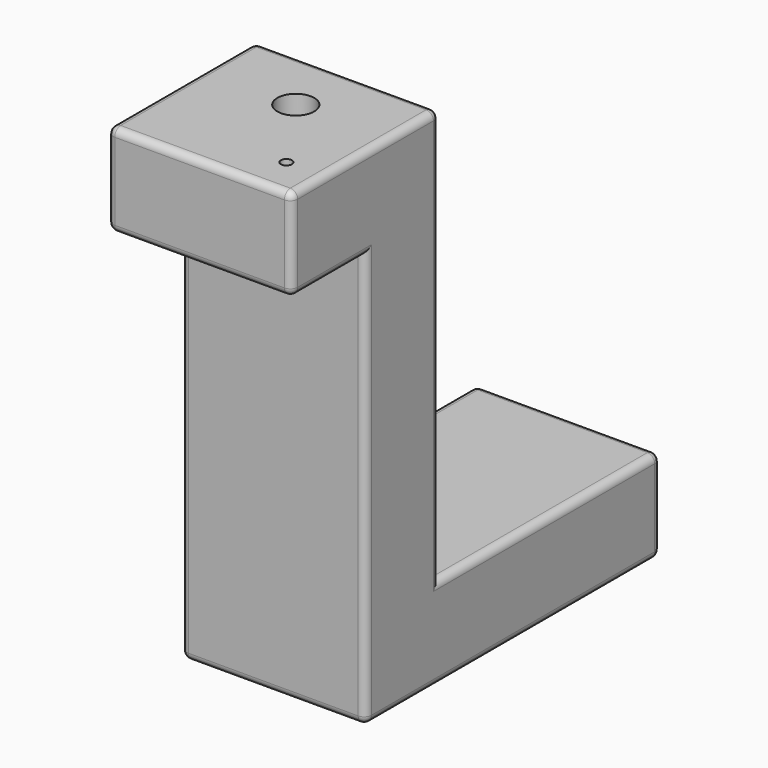
from build123d import *

# Parameters (mm, degrees)
F1_DEPTH      = 6.35
F1_DEPTH_BACK = 6.35
F2_R          = 0.508
F3_T1_DEPTH   = 7.112
F3_T3_DEPTH   = 7.62
F3_T5_DEPTH   = 28.0222646616
F3_T7_DEPTH   = 29.8002646616
F3_T9_DEPTH   = 27.94
F3_T11_DEPTH  = 20.32
F3_T13_DEPTH  = 8.89
F3_S17_W      = 0.508
F3_S17_H      = 0.508
F3_T18_DEPTH  = 0.508
F3_S23_W      = 0.508
F3_S23_H      = 0.508
F3_T24_DEPTH  = 0.508
F3_T31_DEPTH  = 8.89
F3_T35_DEPTH  = 31.0702646616
F3_T42_DEPTH  = 29.2922646616
F3_T46_DEPTH  = 21.59
F4_T1_DEPTH   = 28.0222646616
F4_T3_DEPTH   = 11.684
F4_T5_DEPTH   = 5.334
F4_T7_DEPTH   = 26.162
F4_T9_DEPTH   = 29.8002646616
F4_T11_DEPTH  = 18.542
F4_T13_DEPTH  = 7.62
F4_T15_DEPTH  = 7.112
F4_S19_W      = 0.508
F4_S19_H      = 0.508
F4_T20_DEPTH  = 0.508
F4_S25_W      = 0.508
F4_S25_H      = 0.508
F4_T26_DEPTH  = 0.508
F4_S31_W      = 0.508
F4_S31_H      = 0.508
F4_T32_DEPTH  = 0.508
F4_S37_W      = 0.508
F4_S37_H      = 0.508
F4_T38_DEPTH  = 0.508
F4_S43_W      = 0.508
F4_S43_H      = 0.508
F4_T44_DEPTH  = 0.508
F4_S49_W      = 0.508
F4_S49_H      = 0.508
F4_T50_DEPTH  = 0.508
F4_T57_DEPTH  = 19.812
F4_T61_DEPTH  = 29.2922646616
F4_T68_DEPTH  = 31.0702646616
F4_T72_DEPTH  = 8.89
F5_T1_DEPTH   = 11.684
F5_S5_W       = 0.508
F5_S5_H       = 0.508
F5_T6_DEPTH   = 0.508
F5_S11_W      = 0.508
F5_S11_H      = 0.508
F5_T12_DEPTH  = 0.508
F6_T1_DEPTH   = 11.684
F6_S5_W       = 0.508
F6_S5_H       = 0.508
F6_T6_DEPTH   = 0.508
F6_S11_W      = 0.508
F6_S11_H      = 0.508
F6_T12_DEPTH  = 0.508
F8_D          = 2.54
F8_DEPTH      = 3.175
F8_TIP        = 0.7630929862
F10_D         = 0.762


# Not quite as in the source:
# - a fillet or chamfer that OpenCascade refuses, or shapes differently, is made with other operations: its cross-section is extruded or revolved along the edge and cut away or added


with BuildPart() as f1:
    # F0 (on Right) → F1 (new body, two sides)
    with BuildSketch(Plane.YZ) as f1_sk:
        Polygon((-10.7051408962, 24.1749497761), (-23.4051408962, 24.1749497761), (-23.4051408962, 17.8249497761), (-17.0551408962, 17.8249497761), (-17.0551408962, -10.7053148855), (8.3448591038, -10.7053148855), (8.3448591038, -4.3553148855), (-10.7051408962, -4.3553148855), align=None)
    extrude(amount=F1_DEPTH)
    extrude(f1_sk.sketch, amount=-F1_DEPTH_BACK)

    # F2
    f2_edges = [f1.edges().sort_by_distance(p)[0] for p in [
        (0, -23.405141, 24.17495),
        (6.35, -17.055141, 24.17495),
        (0, -10.705141, 24.17495),
        (-6.35, -17.055141, 24.17495),
    ]]
    fillet(f2_edges, radius=F2_R)

    # F3: fillet of radius 0.508 on 7 edges, made by hand

    # F3_s2 → F3_t1 (cut)
    with BuildSketch(Plane.XY.offset(16.5549497761)):
        with BuildLine():
            ThreePointArc((6.35, -22.8971408962), (6.2012102448, -23.256351141), (5.842, -23.4051408962))
            Line((5.842, -23.4051408962), (6.35, -23.4051408962))
            Line((6.35, -23.4051408962), (6.35, -22.8971408962))
        make_face()
    extrude(amount=F3_T1_DEPTH, mode=Mode.SUBTRACT)

    # F3_s4 → F3_t3 (cut)
    with BuildSketch(Plane.XZ.offset(17.0551408962)):
        with BuildLine():
            ThreePointArc((6.35, 18.3329497761), (6.2012102448, 17.9737395313), (5.842, 17.8249497761))
            Line((5.842, 17.8249497761), (6.35, 17.8249497761))
            Line((6.35, 17.8249497761), (6.35, 18.3329497761))
        make_face()
    extrude(amount=F3_T3_DEPTH, mode=Mode.SUBTRACT)

    # F3_s6 → F3_t5 (cut)
    with BuildSketch(Plane.XY.offset(-4.3553148855)):
        with BuildLine():
            ThreePointArc((5.842, -10.7051408962), (6.2012102448, -10.8539306514), (6.35, -11.2131408962))
            Line((6.35, -11.2131408962), (6.35, -10.7051408962))
            Line((6.35, -10.7051408962), (5.842, -10.7051408962))
        make_face()
    extrude(amount=F3_T5_DEPTH, mode=Mode.SUBTRACT)

    # F3_s8 → F3_t7 (cut)
    with BuildSketch(Plane.XY.offset(-11.9753148855)):
        with BuildLine():
            ThreePointArc((6.35, -16.5471408962), (6.2012102448, -16.906351141), (5.842, -17.0551408962))
            Line((5.842, -17.0551408962), (6.35, -17.0551408962))
            Line((6.35, -17.0551408962), (6.35, -16.5471408962))
        make_face()
    extrude(amount=F3_T7_DEPTH, mode=Mode.SUBTRACT)

    # F3_s10 → F3_t9 (cut)
    with BuildSketch(Plane.XZ.offset(-9.6148591038)):
        with BuildLine():
            ThreePointArc((6.35, -10.1973148855), (6.2012102448, -10.5565251304), (5.842, -10.7053148855))
            Line((5.842, -10.7053148855), (6.35, -10.7053148855))
            Line((6.35, -10.7053148855), (6.35, -10.1973148855))
        make_face()
    extrude(amount=F3_T9_DEPTH, mode=Mode.SUBTRACT)

    # F3_s12 → F3_t11 (cut)
    with BuildSketch(Plane.XZ.offset(-9.6148591038)):
        with BuildLine():
            ThreePointArc((6.35, -4.8633148855), (6.2012102448, -4.5041046407), (5.842, -4.3553148855))
            Line((5.842, -4.3553148855), (6.35, -4.3553148855))
            Line((6.35, -4.3553148855), (6.35, -4.8633148855))
        make_face()
    extrude(amount=F3_T11_DEPTH, mode=Mode.SUBTRACT)

    # F3_s14 → F3_t13 (cut)
    with BuildSketch(Plane.XY.offset(-11.9753148855)):
        with BuildLine():
            ThreePointArc((6.35, 7.8368591038), (6.2012102448, 8.1960693486), (5.842, 8.3448591038))
            Line((5.842, 8.3448591038), (6.35, 8.3448591038))
            Line((6.35, 8.3448591038), (6.35, 7.8368591038))
        make_face()
    extrude(amount=F3_T13_DEPTH, mode=Mode.SUBTRACT)


with BuildPart() as f3_tool16:
    # F3_s17 → F3_t18 (new body)
    with BuildSketch(Plane.XZ.offset(11.2131408962)):
        with Locations((6.096, 23.9209497761)):
            Rectangle(F3_S17_W, F3_S17_H)
    extrude(amount=-F3_T18_DEPTH)

    # F3_s19 → F3_t20 (revolve, cut)
    with BuildSketch(Plane(origin=(5.842, -11.2131408962, 23.6669497761), x_dir=(-0.7071067812, 0, -0.7071067812), z_dir=(0.7071067812, 0, -0.7071067812))):
        with BuildLine():
            ThreePointArc((0, -0.508), (0.508, 0), (0, 0.508))
            Line((0, 0.508), (0, -0.508))
        make_face()
    revolve(axis=Axis((5.842, -11.2131408962, 23.6669497761), (0, 1, 0)), mode=Mode.SUBTRACT)


with BuildPart() as f1_1:
    add(f1.part)

    # F3_t15: cut F3_tool16
    add(f3_tool16.part, mode=Mode.SUBTRACT)


with BuildPart() as f3_tool22:
    # F3_s23 → F3_t24 (new body)
    with BuildSketch(Plane.YZ.offset(5.842)):
        with Locations((-23.1511408962, 23.9209497761)):
            Rectangle(F3_S23_W, F3_S23_H)
    extrude(amount=F3_T24_DEPTH)

    # F3_s25 → F3_t26 (revolve, cut)
    with BuildSketch(Plane(origin=(5.842, -22.8971408962, 23.6669497761), x_dir=(0, 0.7071067812, -0.7071067812), z_dir=(0, -0.7071067812, -0.7071067812))):
        with BuildLine():
            ThreePointArc((0, -0.508), (0.508, 0), (0, 0.508))
            Line((0, 0.508), (0, -0.508))
        make_face()
    revolve(axis=Axis((5.842, -22.8971408962, 23.6669497761), (1, 0, 0)), mode=Mode.SUBTRACT)


with BuildPart() as f1_2:
    add(f1_1.part)

    # F3_t21: cut F3_tool22
    add(f3_tool22.part, mode=Mode.SUBTRACT)


with BuildPart() as f3_tool29:
    # F3_s30 → F3_t31 (new body)
    with BuildSketch(Plane.XZ.offset(24.6751408962)):
        with BuildLine():
            ThreePointArc((6.35, 18.3329497761), (6.2012102448, 17.9737395313), (5.842, 17.8249497761))
            Line((5.842, 17.8249497761), (6.35, 17.8249497761))
            Line((6.35, 17.8249497761), (6.35, 18.3329497761))
        make_face()
    extrude(amount=-F3_T31_DEPTH)

    split(bisect_by=Plane.XZ.offset(17.0551408962), keep=Keep.BOTTOM)


with BuildPart() as f3_tool33:
    # F3_s34 → F3_t35 (new body)
    with BuildSketch(Plane.XY.offset(19.0949497761)):
        with BuildLine():
            ThreePointArc((6.35, -16.5471408962), (6.2012102448, -16.906351141), (5.842, -17.0551408962))
            Line((5.842, -17.0551408962), (6.35, -17.0551408962))
            Line((6.35, -17.0551408962), (6.35, -16.5471408962))
        make_face()
    extrude(amount=-F3_T35_DEPTH)

    split(bisect_by=Plane.XY.offset(17.8249497761), keep=Keep.TOP)


with BuildPart() as f3_tool29_1:
    add(f3_tool29.part)

    # F3_t37: intersect F3_tool33
    add(f3_tool33.part, mode=Mode.INTERSECT)


with BuildPart() as f1_3:
    add(f1_2.part)

    # F3_t27: cut F3_tool29
    add(f3_tool29_1.part, mode=Mode.SUBTRACT)


with BuildPart() as f3_tool40:
    # F3_s41 → F3_t42 (new body)
    with BuildSketch(Plane.XY.offset(-5.6253148855)):
        with BuildLine():
            ThreePointArc((5.842, -10.7051408962), (6.2012102448, -10.8539306514), (6.35, -11.2131408962))
            Line((6.35, -11.2131408962), (6.35, -10.7051408962))
            Line((6.35, -10.7051408962), (5.842, -10.7051408962))
        make_face()
    extrude(amount=F3_T42_DEPTH)

    split(bisect_by=Plane.XY.offset(-4.3553148855), keep=Keep.BOTTOM)


with BuildPart() as f3_tool44:
    # F3_s45 → F3_t46 (new body)
    with BuildSketch(Plane.XZ.offset(-9.6148591038)):
        with BuildLine():
            ThreePointArc((6.35, -4.8633148855), (6.2012102448, -4.5041046407), (5.842, -4.3553148855))
            Line((5.842, -4.3553148855), (6.35, -4.3553148855))
            Line((6.35, -4.3553148855), (6.35, -4.8633148855))
        make_face()
    extrude(amount=F3_T46_DEPTH)

    split(bisect_by=Plane.XZ.offset(10.7051408962), keep=Keep.TOP)


with BuildPart() as f3_tool40_1:
    add(f3_tool40.part)

    # F3_t48: intersect F3_tool44
    add(f3_tool44.part, mode=Mode.INTERSECT)


with BuildPart() as f1_4:
    add(f1_3.part)

    # F3_t38: cut F3_tool40
    add(f3_tool40_1.part, mode=Mode.SUBTRACT)

    # F4: fillet of radius 0.508 on 9 edges, made by hand

    # F4_s2 → F4_t1 (cut)
    with BuildSketch(Plane.XY.offset(-4.3553148855)):
        with BuildLine():
            ThreePointArc((-5.842, -10.7051408962), (-6.2012102448, -10.8539306514), (-6.35, -11.2131408962))
            Line((-6.35, -11.2131408962), (-6.35, -10.7051408962))
            Line((-6.35, -10.7051408962), (-5.842, -10.7051408962))
        make_face()
    extrude(amount=F4_T1_DEPTH, mode=Mode.SUBTRACT)

    # F4_s4 → F4_t3 (cut)
    with BuildSketch(Plane.YZ.offset(-5.842)):
        with BuildLine():
            ThreePointArc((7.8368591038, -4.3553148855), (8.1960693486, -4.5041046407), (8.3448591038, -4.8633148855))
            Line((8.3448591038, -4.8633148855), (8.3448591038, -4.3553148855))
            Line((8.3448591038, -4.3553148855), (7.8368591038, -4.3553148855))
        make_face()
        with BuildLine():
            ThreePointArc((7.8368591038, -10.7053148855), (8.1960693486, -10.5565251304), (8.3448591038, -10.1973148855))
            Line((8.3448591038, -10.1973148855), (8.3448591038, -10.7053148855))
            Line((8.3448591038, -10.7053148855), (7.8368591038, -10.7053148855))
        make_face()
    extrude(amount=F4_T3_DEPTH, mode=Mode.SUBTRACT)

    # F4_s6 → F4_t5 (cut)
    with BuildSketch(Plane.XY.offset(-10.1973148855)):
        with BuildLine():
            ThreePointArc((-6.35, 7.8368591038), (-6.2012102448, 8.1960693486), (-5.842, 8.3448591038))
            Line((-5.842, 8.3448591038), (-6.35, 8.3448591038))
            Line((-6.35, 8.3448591038), (-6.35, 7.8368591038))
        make_face()
    extrude(amount=F4_T5_DEPTH, mode=Mode.SUBTRACT)

    # F4_s8 → F4_t7 (cut)
    with BuildSketch(Plane.XZ.offset(-7.8368591038)):
        with BuildLine():
            ThreePointArc((-5.842, -10.7053148855), (-6.2012102448, -10.5565251304), (-6.35, -10.1973148855))
            Line((-6.35, -10.1973148855), (-6.35, -10.7053148855))
            Line((-6.35, -10.7053148855), (-5.842, -10.7053148855))
        make_face()
    extrude(amount=F4_T7_DEPTH, mode=Mode.SUBTRACT)

    # F4_s10 → F4_t9 (cut)
    with BuildSketch(Plane.XY.offset(-11.9753148855)):
        with BuildLine():
            ThreePointArc((-5.842, -17.0551408962), (-6.2012102448, -16.906351141), (-6.35, -16.5471408962))
            Line((-6.35, -16.5471408962), (-6.35, -17.0551408962))
            Line((-6.35, -17.0551408962), (-5.842, -17.0551408962))
        make_face()
    extrude(amount=F4_T9_DEPTH, mode=Mode.SUBTRACT)

    # F4_s12 → F4_t11 (cut)
    with BuildSketch(Plane.XZ.offset(-7.8368591038)):
        with BuildLine():
            ThreePointArc((-5.842, -4.3553148855), (-6.2012102448, -4.5041046407), (-6.35, -4.8633148855))
            Line((-6.35, -4.8633148855), (-6.35, -4.3553148855))
            Line((-6.35, -4.3553148855), (-5.842, -4.3553148855))
        make_face()
    extrude(amount=F4_T11_DEPTH, mode=Mode.SUBTRACT)

    # F4_s14 → F4_t13 (cut)
    with BuildSketch(Plane.XZ.offset(17.0551408962)):
        with BuildLine():
            ThreePointArc((-5.842, 17.8249497761), (-6.2012102448, 17.9737395313), (-6.35, 18.3329497761))
            Line((-6.35, 18.3329497761), (-6.35, 17.8249497761))
            Line((-6.35, 17.8249497761), (-5.842, 17.8249497761))
        make_face()
    extrude(amount=F4_T13_DEPTH, mode=Mode.SUBTRACT)

    # F4_s16 → F4_t15 (cut)
    with BuildSketch(Plane.XY.offset(16.5549497761)):
        with BuildLine():
            ThreePointArc((-5.842, -23.4051408962), (-6.2012102448, -23.256351141), (-6.35, -22.8971408962))
            Line((-6.35, -22.8971408962), (-6.35, -23.4051408962))
            Line((-6.35, -23.4051408962), (-5.842, -23.4051408962))
        make_face()
    extrude(amount=F4_T15_DEPTH, mode=Mode.SUBTRACT)


with BuildPart() as f4_tool18:
    # F4_s19 → F4_t20 (new body)
    with BuildSketch(Plane.XZ.offset(22.8971408962)):
        with Locations((-6.096, 23.9209497761)):
            Rectangle(F4_S19_W, F4_S19_H)
    extrude(amount=F4_T20_DEPTH)

    # F4_s21 → F4_t22 (revolve, cut)
    with BuildSketch(Plane(origin=(-5.842, -22.8971408962, 23.6669497761), x_dir=(0.7071067812, 0, -0.7071067812), z_dir=(-0.7071067812, 0, -0.7071067812))):
        with BuildLine():
            ThreePointArc((0, -0.508), (0.508, 0), (0, 0.508))
            Line((0, 0.508), (0, -0.508))
        make_face()
    revolve(axis=Axis((-5.842, -22.8971408962, 23.6669497761), (0, -1, 0)), mode=Mode.SUBTRACT)


with BuildPart() as f1_5:
    add(f1_4.part)

    # F4_t17: cut F4_tool18
    add(f4_tool18.part, mode=Mode.SUBTRACT)


with BuildPart() as f4_tool24:
    # F4_s25 → F4_t26 (new body)
    with BuildSketch(Plane.XY.offset(-10.1973148855)):
        with Locations((6.096, 8.0908591038)):
            Rectangle(F4_S25_W, F4_S25_H)
    extrude(amount=-F4_T26_DEPTH)

    # F4_s27 → F4_t28 (revolve, cut)
    with BuildSketch(Plane(origin=(5.842, 7.8368591038, -10.1973148855), x_dir=(-0.7071067812, -0.7071067812, 0), z_dir=(0.7071067812, -0.7071067812, 0))):
        with BuildLine():
            ThreePointArc((0, -0.508), (0.508, 0), (0, 0.508))
            Line((0, 0.508), (0, -0.508))
        make_face()
    revolve(axis=Axis((5.842, 7.8368591038, -10.1973148855), (0, 0, -1)), mode=Mode.SUBTRACT)


with BuildPart() as f1_6:
    add(f1_5.part)

    # F4_t23: cut F4_tool24
    add(f4_tool24.part, mode=Mode.SUBTRACT)


with BuildPart() as f4_tool30:
    # F4_s31 → F4_t32 (new body)
    with BuildSketch(Plane.XY.offset(-4.8633148855)):
        with Locations((6.096, 8.0908591038)):
            Rectangle(F4_S31_W, F4_S31_H)
    extrude(amount=F4_T32_DEPTH)

    # F4_s33 → F4_t34 (revolve, cut)
    with BuildSketch(Plane(origin=(5.842, 7.8368591038, -4.8633148855), x_dir=(-0.7071067812, -0.7071067812, 0), z_dir=(-0.7071067812, 0.7071067812, 0))):
        with BuildLine():
            ThreePointArc((0, -0.508), (0.508, 0), (0, 0.508))
            Line((0, 0.508), (0, -0.508))
        make_face()
    revolve(axis=Axis((5.842, 7.8368591038, -4.8633148855), (0, 0, 1)), mode=Mode.SUBTRACT)


with BuildPart() as f1_7:
    add(f1_6.part)

    # F4_t29: cut F4_tool30
    add(f4_tool30.part, mode=Mode.SUBTRACT)


with BuildPart() as f4_tool36:
    # F4_s37 → F4_t38 (new body)
    with BuildSketch(Plane.XZ.offset(11.2131408962)):
        with Locations((-6.096, 23.9209497761)):
            Rectangle(F4_S37_W, F4_S37_H)
    extrude(amount=-F4_T38_DEPTH)

    # F4_s39 → F4_t40 (revolve, cut)
    with BuildSketch(Plane(origin=(-5.842, -11.2131408962, 23.6669497761), x_dir=(0.7071067812, 0, -0.7071067812), z_dir=(0.7071067812, 0, 0.7071067812))):
        with BuildLine():
            ThreePointArc((0, -0.508), (0.508, 0), (0, 0.508))
            Line((0, 0.508), (0, -0.508))
        make_face()
    revolve(axis=Axis((-5.842, -11.2131408962, 23.6669497761), (0, 1, 0)), mode=Mode.SUBTRACT)


with BuildPart() as f1_8:
    add(f1_7.part)

    # F4_t35: cut F4_tool36
    add(f4_tool36.part, mode=Mode.SUBTRACT)


with BuildPart() as f4_tool42:
    # F4_s43 → F4_t44 (new body)
    with BuildSketch(Plane.XY.offset(-4.8633148855)):
        with Locations((-6.096, 8.0908591038)):
            Rectangle(F4_S43_W, F4_S43_H)
    extrude(amount=F4_T44_DEPTH)

    # F4_s45 → F4_t46 (revolve, cut)
    with BuildSketch(Plane(origin=(-5.842, 7.8368591038, -4.8633148855), x_dir=(0.7071067812, -0.7071067812, 0), z_dir=(-0.7071067812, -0.7071067812, 0))):
        with BuildLine():
            ThreePointArc((0, -0.508), (0.508, 0), (0, 0.508))
            Line((0, 0.508), (0, -0.508))
        make_face()
    revolve(axis=Axis((-5.842, 7.8368591038, -4.8633148855), (0, 0, 1)), mode=Mode.SUBTRACT)


with BuildPart() as f1_9:
    add(f1_8.part)

    # F4_t41: cut F4_tool42
    add(f4_tool42.part, mode=Mode.SUBTRACT)


with BuildPart() as f4_tool48:
    # F4_s49 → F4_t50 (new body)
    with BuildSketch(Plane.XY.offset(-10.1973148855)):
        with Locations((-6.096, 8.0908591038)):
            Rectangle(F4_S49_W, F4_S49_H)
    extrude(amount=-F4_T50_DEPTH)

    # F4_s51 → F4_t52 (revolve, cut)
    with BuildSketch(Plane(origin=(-5.842, 7.8368591038, -10.1973148855), x_dir=(0.7071067812, -0.7071067812, 0), z_dir=(0.7071067812, 0.7071067812, 0))):
        with BuildLine():
            ThreePointArc((0, -0.508), (0.508, 0), (0, 0.508))
            Line((0, 0.508), (0, -0.508))
        make_face()
    revolve(axis=Axis((-5.842, 7.8368591038, -10.1973148855), (0, 0, -1)), mode=Mode.SUBTRACT)


with BuildPart() as f1_10:
    add(f1_9.part)

    # F4_t47: cut F4_tool48
    add(f4_tool48.part, mode=Mode.SUBTRACT)


with BuildPart() as f4_tool55:
    # F4_s56 → F4_t57 (new body)
    with BuildSketch(Plane.XZ.offset(-7.8368591038)):
        with BuildLine():
            ThreePointArc((-5.842, -4.3553148855), (-6.2012102448, -4.5041046407), (-6.35, -4.8633148855))
            Line((-6.35, -4.8633148855), (-6.35, -4.3553148855))
            Line((-6.35, -4.3553148855), (-5.842, -4.3553148855))
        make_face()
    extrude(amount=F4_T57_DEPTH)

    split(bisect_by=Plane.XZ.offset(10.7051408962), keep=Keep.TOP)


with BuildPart() as f4_tool59:
    # F4_s60 → F4_t61 (new body)
    with BuildSketch(Plane.XY.offset(-5.6253148855)):
        with BuildLine():
            ThreePointArc((-5.842, -10.7051408962), (-6.2012102448, -10.8539306514), (-6.35, -11.2131408962))
            Line((-6.35, -11.2131408962), (-6.35, -10.7051408962))
            Line((-6.35, -10.7051408962), (-5.842, -10.7051408962))
        make_face()
    extrude(amount=F4_T61_DEPTH)

    split(bisect_by=Plane.XY.offset(-4.3553148855), keep=Keep.BOTTOM)


with BuildPart() as f4_tool55_1:
    add(f4_tool55.part)

    # F4_t63: intersect F4_tool59
    add(f4_tool59.part, mode=Mode.INTERSECT)


with BuildPart() as f1_11:
    add(f1_10.part)

    # F4_t53: cut F4_tool55
    add(f4_tool55_1.part, mode=Mode.SUBTRACT)


with BuildPart() as f4_tool66:
    # F4_s67 → F4_t68 (new body)
    with BuildSketch(Plane.XY.offset(19.0949497761)):
        with BuildLine():
            ThreePointArc((-5.842, -17.0551408962), (-6.2012102448, -16.906351141), (-6.35, -16.5471408962))
            Line((-6.35, -16.5471408962), (-6.35, -17.0551408962))
            Line((-6.35, -17.0551408962), (-5.842, -17.0551408962))
        make_face()
    extrude(amount=-F4_T68_DEPTH)

    split(bisect_by=Plane.XY.offset(17.8249497761), keep=Keep.TOP)


with BuildPart() as f4_tool70:
    # F4_s71 → F4_t72 (new body)
    with BuildSketch(Plane.XZ.offset(24.6751408962)):
        with BuildLine():
            ThreePointArc((-5.842, 17.8249497761), (-6.2012102448, 17.9737395313), (-6.35, 18.3329497761))
            Line((-6.35, 18.3329497761), (-6.35, 17.8249497761))
            Line((-6.35, 17.8249497761), (-5.842, 17.8249497761))
        make_face()
    extrude(amount=-F4_T72_DEPTH)

    split(bisect_by=Plane.XZ.offset(17.0551408962), keep=Keep.BOTTOM)


with BuildPart() as f4_tool66_1:
    add(f4_tool66.part)

    # F4_t74: intersect F4_tool70
    add(f4_tool70.part, mode=Mode.INTERSECT)


with BuildPart() as f1_12:
    add(f1_11.part)

    # F4_t64: cut F4_tool66
    add(f4_tool66_1.part, mode=Mode.SUBTRACT)

    # F5: fillet of radius 0.508 on 1 edges, made by hand

    # F5_s2 → F5_t1 (cut)
    with BuildSketch(Plane.YZ.offset(-5.842)):
        with BuildLine():
            ThreePointArc((-17.0551408962, -10.1973148855), (-16.906351141, -10.5565251304), (-16.5471408962, -10.7053148855))
            Line((-16.5471408962, -10.7053148855), (-17.0551408962, -10.7053148855))
            Line((-17.0551408962, -10.7053148855), (-17.0551408962, -10.1973148855))
        make_face()
    extrude(amount=F5_T1_DEPTH, mode=Mode.SUBTRACT)


with BuildPart() as f5_tool4:
    # F5_s5 → F5_t6 (new body)
    with BuildSketch(Plane.XZ.offset(16.5471408962)):
        with Locations((-6.096, -10.4513148855)):
            Rectangle(F5_S5_W, F5_S5_H)
    extrude(amount=F5_T6_DEPTH)

    # F5_s7 → F5_t8 (revolve, cut)
    with BuildSketch(Plane(origin=(-5.842, -16.5471408962, -10.1973148855), x_dir=(0.7071067812, 0, 0.7071067812), z_dir=(0.7071067812, 0, -0.7071067812))):
        with BuildLine():
            ThreePointArc((0, -0.508), (0.508, 0), (0, 0.508))
            Line((0, 0.508), (0, -0.508))
        make_face()
    revolve(axis=Axis((-5.842, -16.5471408962, -10.1973148855), (0, -1, 0)), mode=Mode.SUBTRACT)


with BuildPart() as f1_13:
    add(f1_12.part)

    # F5_t3: cut F5_tool4
    add(f5_tool4.part, mode=Mode.SUBTRACT)


with BuildPart() as f5_tool10:
    # F5_s11 → F5_t12 (new body)
    with BuildSketch(Plane.XZ.offset(16.5471408962)):
        with Locations((6.096, -10.4513148855)):
            Rectangle(F5_S11_W, F5_S11_H)
    extrude(amount=F5_T12_DEPTH)

    # F5_s13 → F5_t14 (revolve, cut)
    with BuildSketch(Plane(origin=(5.842, -16.5471408962, -10.1973148855), x_dir=(-0.7071067812, 0, 0.7071067812), z_dir=(0.7071067812, 0, 0.7071067812))):
        with BuildLine():
            ThreePointArc((0, -0.508), (0.508, 0), (0, 0.508))
            Line((0, 0.508), (0, -0.508))
        make_face()
    revolve(axis=Axis((5.842, -16.5471408962, -10.1973148855), (0, -1, 0)), mode=Mode.SUBTRACT)


with BuildPart() as f1_14:
    add(f1_13.part)

    # F5_t9: cut F5_tool10
    add(f5_tool10.part, mode=Mode.SUBTRACT)

    # F6: fillet of radius 0.508 on 1 edges, made by hand

    # F6_s2 → F6_t1 (cut)
    with BuildSketch(Plane.YZ.offset(-5.842)):
        with BuildLine():
            ThreePointArc((-23.4051408962, 18.3329497761), (-23.256351141, 17.9737395313), (-22.8971408962, 17.8249497761))
            Line((-22.8971408962, 17.8249497761), (-23.4051408962, 17.8249497761))
            Line((-23.4051408962, 17.8249497761), (-23.4051408962, 18.3329497761))
        make_face()
    extrude(amount=F6_T1_DEPTH, mode=Mode.SUBTRACT)


with BuildPart() as f6_tool4:
    # F6_s5 → F6_t6 (new body)
    with BuildSketch(Plane.XZ.offset(22.8971408962)):
        with Locations((-6.096, 18.0789497761)):
            Rectangle(F6_S5_W, F6_S5_H)
    extrude(amount=F6_T6_DEPTH)

    # F6_s7 → F6_t8 (revolve, cut)
    with BuildSketch(Plane(origin=(-5.842, -22.8971408962, 18.3329497761), x_dir=(0.7071067812, 0, 0.7071067812), z_dir=(0.7071067812, 0, -0.7071067812))):
        with BuildLine():
            ThreePointArc((0, -0.508), (0.508, 0), (0, 0.508))
            Line((0, 0.508), (0, -0.508))
        make_face()
    revolve(axis=Axis((-5.842, -22.8971408962, 18.3329497761), (0, -1, 0)), mode=Mode.SUBTRACT)


with BuildPart() as f1_15:
    add(f1_14.part)

    # F6_t3: cut F6_tool4
    add(f6_tool4.part, mode=Mode.SUBTRACT)


with BuildPart() as f6_tool10:
    # F6_s11 → F6_t12 (new body)
    with BuildSketch(Plane.XZ.offset(22.8971408962)):
        with Locations((6.096, 18.0789497761)):
            Rectangle(F6_S11_W, F6_S11_H)
    extrude(amount=F6_T12_DEPTH)

    # F6_s13 → F6_t14 (revolve, cut)
    with BuildSketch(Plane(origin=(5.842, -22.8971408962, 18.3329497761), x_dir=(-0.7071067812, 0, 0.7071067812), z_dir=(0.7071067812, 0, 0.7071067812))):
        with BuildLine():
            ThreePointArc((0, -0.508), (0.508, 0), (0, 0.508))
            Line((0, 0.508), (0, -0.508))
        make_face()
    revolve(axis=Axis((5.842, -22.8971408962, 18.3329497761), (0, -1, 0)), mode=Mode.SUBTRACT)


with BuildPart() as f1_16:
    add(f1_15.part)

    # F6_t9: cut F6_tool10
    add(f6_tool10.part, mode=Mode.SUBTRACT)

    # F8
    with Locations(Plane.XY.offset(24.1749497761)):
        with Locations((0, -15.1246003807)):
            Hole(F8_D / 2, depth=F8_DEPTH)
            with Locations((0, 0, -(F8_DEPTH + F8_TIP / 2))):  # 118° drill point
                Cone(0, F8_D / 2, F8_TIP, mode=Mode.SUBTRACT)

    # F10 (through all)
    with Locations(Plane.XY.offset(24.1749497761)):
        with Locations((3.7932256237, -20.6758901477)):
            Hole(F10_D / 2)


solid = f1_16.part
